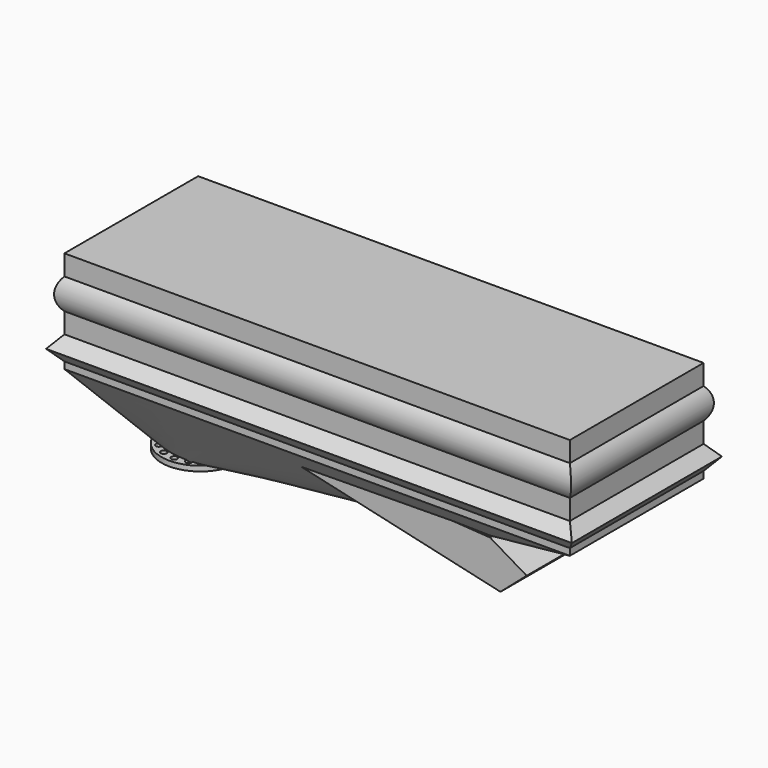
from build123d import *

# Parameters (mm, degrees)
F0_W       = 2580
F0_H       = 500
F1_DEPTH   = 475
F3_DEPTH   = 950
F5_DEPTH   = 2500
F1_FACE1_W = 2480
F1_FACE1_H = 820
F7_R       = 190
F7_R_2     = 15
F7_R_3     = 125
F9_DEPTH   = 25
F11_DEPTH  = 350


# Not quite as in the source:
# - the arcs of a loft's sections are written as splines that run evenly, so that the points pair up as in the source's solid


with BuildPart() as f1:
    # F0 (on Front) → F1 (new body, symmetric)
    with BuildSketch(Plane.XZ):
        Rectangle(F0_W, F0_H)
    extrude(amount=F1_DEPTH, both=True)

    # F2 (on face) → F3 (cut, through all)
    with BuildSketch(Plane.XZ.offset(475)):
        with BuildLine():
            Line((-1240, 150.2039159699), (-1240, 250))
            Line((-1240, 250), (-1240, 361.6854846478))
            Line((-1240, 361.6854846478), (-1458.3188199997, 361.6854846478))
            Line((-1458.3188199997, 361.6854846478), (-1458.3188199997, -342.266112566))
            Line((-1458.3188199997, -342.266112566), (-1240, -342.266112566))
            Line((-1240, -342.266112566), (-1240, -216.8733626604))
            Line((-1240, -216.8733626604), (-1290, -158.3347233453))
            Line((-1290, -158.3347233453), (-1240, -99.7960840301))
            Line((-1240, -99.7960840301), (-1240, 0))
            ThreePointArc((-1240, 0), (-1268.1875295389, 75.1019579849), (-1240, 150.2039159699))
        make_face()
        with BuildLine():
            ThreePointArc((1240, 150.2039159699), (1268.1875295389, 75.1019579849), (1240, 0))
            Line((1240, 0), (1240, -99.7960840301))
            Line((1240, -99.7960840301), (1290, -158.3347233453))
            Line((1290, -158.3347233453), (1240, -216.8733626604))
            Line((1240, -216.8733626604), (1240, -342.266112566))
            Line((1240, -342.266112566), (1458.3188199997, -342.266112566))
            Line((1458.3188199997, -342.266112566), (1458.3188199997, 361.6854846478))
            Line((1458.3188199997, 361.6854846478), (1240, 361.6854846478))
            Line((1240, 361.6854846478), (1240, 250))
            Line((1240, 250), (1240, 150.2039159699))
        make_face()
    extrude(amount=-F3_DEPTH, mode=Mode.SUBTRACT)

    # F4 (on Right) → F5 (cut, symmetric)
    with BuildSketch(Plane.YZ):
        with BuildLine():
            Line((-410, 150.2039159699), (-410, 250))
            Line((-410, 250), (-410, 357.733887434))
            Line((-410, 357.733887434), (-610, 357.733887434))
            Line((-610, 357.733887434), (-610, -342.266112566))
            Line((-610, -342.266112566), (-410, -342.266112566))
            Line((-410, -342.266112566), (-410, -216.8733626604))
            Line((-410, -216.8733626604), (-460, -158.3347233453))
            Line((-460, -158.3347233453), (-410, -99.7960840301))
            Line((-410, -99.7960840301), (-410, 0))
            ThreePointArc((-410, 0), (-438.1766354959, 75.1019579849), (-410, 150.2039159699))
        make_face()
        with BuildLine():
            ThreePointArc((410, 150.2039159699), (438.1766354959, 75.1019579849), (410, 0))
            Line((410, 0), (410, -99.7960840301))
            Line((410, -99.7960840301), (460, -158.3347233453))
            Line((460, -158.3347233453), (410, -216.8733626604))
            Line((410, -216.8733626604), (410, -342.266112566))
            Line((410, -342.266112566), (610, -342.266112566))
            Line((610, -342.266112566), (610, 357.733887434))
            Line((610, 357.733887434), (410, 357.733887434))
            Line((410, 357.733887434), (410, 250))
            Line((410, 250), (410, 150.2039159699))
        make_face()
    extrude(amount=F5_DEPTH, both=True, mode=Mode.SUBTRACT)

    # F7 (on offset) → F8 section 0
    with BuildSketch(Plane(origin=(0, 0, -650), x_dir=(1, 0, 0), z_dir=(0, 0, -1))):
        with BuildLine():
            add(Edge.make_bspline(
                [(-980.6526777918, 96.3350970343), (-986.9577951485, 91.1218414637), (-992.749308438, 85.2877302997), (-1003.0831296115, 72.6014268955), (-1007.6251819714, 65.749548349), (-1015.2854666523, 51.290980207), (-1018.4035095577, 43.6846481281), (-1023.0958773017, 28.0094499136), (-1024.6700861123, 19.9409713782), (-1026.2142118585, 3.6515321678), (-1026.1840906126, -4.5690257187), (-1024.5206344746, -20.8467119114), (-1022.8873407148, -28.9034377196), (-1018.080228379, -44.5438285428), (-1014.9065286684, -52.1271068182), (-1007.1404947661, -66.5291508238), (-1002.5483526049, -73.347560435), (-997.3350970343, -79.6526777918)],
                knots=[0, 0, 0, 0, 0.125, 0.125, 0.25, 0.25, 0.375, 0.375, 0.5, 0.5, 0.625, 0.625, 0.75, 0.75, 0.875, 0.875, 1, 1, 1, 1], degree=3))
            add(Edge.make_bspline(
                [(-997.3350970343, -79.6526777918), (-992.1218414637, -85.9577951485), (-986.2877302997, -91.749308438), (-973.6014268955, -102.0831296115), (-966.749548349, -106.6251819714), (-952.290980207, -114.2854666523), (-944.6846481281, -117.4035095577), (-929.0094499136, -122.0958773017), (-920.9409713782, -123.6700861123), (-904.6515321678, -125.2142118585), (-896.4309742813, -125.1840906126), (-880.1532880886, -123.5206344746), (-872.0965622804, -121.8873407148), (-856.4561714572, -117.080228379), (-848.8728931818, -113.9065286684), (-834.4708491762, -106.1404947661), (-827.652439565, -101.5483526049), (-821.3473222082, -96.3350970343)],
                knots=[0, 0, 0, 0, 0.125, 0.125, 0.25, 0.25, 0.375, 0.375, 0.5, 0.5, 0.625, 0.625, 0.75, 0.75, 0.875, 0.875, 1, 1, 1, 1], degree=3))
            add(Edge.make_bspline(
                [(-821.3473222082, -96.3350970343), (-815.0422048515, -91.1218414637), (-809.250691562, -85.2877302997), (-798.9168703885, -72.6014268955), (-794.3748180286, -65.749548349), (-786.7145333477, -51.290980207), (-783.5964904423, -43.6846481281), (-778.9041226983, -28.0094499136), (-777.3299138877, -19.9409713782), (-775.7857881415, -3.6515321678), (-775.8159093874, 4.5690257187), (-777.4793655254, 20.8467119114), (-779.1126592852, 28.9034377196), (-783.919771621, 44.5438285428), (-787.0934713316, 52.1271068182), (-794.8595052339, 66.5291508238), (-799.4516473951, 73.347560435), (-804.6649029657, 79.6526777918)],
                knots=[0, 0, 0, 0, 0.125, 0.125, 0.25, 0.25, 0.375, 0.375, 0.5, 0.5, 0.625, 0.625, 0.75, 0.75, 0.875, 0.875, 1, 1, 1, 1], degree=3))
            add(Edge.make_bspline(
                [(-804.6649029657, 79.6526777918), (-809.8781585363, 85.9577951485), (-815.7122697003, 91.749308438), (-828.3985731045, 102.0831296115), (-835.250451651, 106.6251819714), (-849.709019793, 114.2854666523), (-857.3153518719, 117.4035095577), (-872.9905500864, 122.0958773017), (-881.0590286218, 123.6700861123), (-897.3484678322, 125.2142118585), (-905.5690257187, 125.1840906126), (-921.8467119114, 123.5206344746), (-929.9034377196, 121.8873407148), (-945.5438285428, 117.080228379), (-953.1271068182, 113.9065286684), (-967.5291508238, 106.1404947661), (-974.347560435, 101.5483526049), (-980.6526777918, 96.3350970343)],
                knots=[0, 0, 0, 0, 0.125, 0.125, 0.25, 0.25, 0.375, 0.375, 0.5, 0.5, 0.625, 0.625, 0.75, 0.75, 0.875, 0.875, 1, 1, 1, 1], degree=3))
        make_face()
    # F1_face1 (on face) → F8 section 1
    with BuildSketch(Plane(origin=(0, 0, -250), x_dir=(1, 0, 0), z_dir=(0, 0, -1))):
        Rectangle(F1_FACE1_W, F1_FACE1_H)
    loft(ruled=True)

    # F10 (on Front) → F11 (join, symmetric)
    with BuildSketch(Plane.XZ):
        Polygon((980.0000190735, -444.9000358582), (800.8000254631, -338.5000228882), (-487.2000217438, -251.700013876), (851.3677120209, -556.3215613365), align=None)
    extrude(amount=F11_DEPTH, both=True)


with BuildPart() as f9:
    # F7 (on offset) → F9 (new body)
    with BuildSketch(Plane(origin=(0, 0, -650), x_dir=(1, 0, 0), z_dir=(0, 0, -1))):
        with Locations((-901, 0)):
            Circle(F7_R)
        with Locations((-1014.1370849898, -113.1370849898)):
            Circle(F7_R_2, mode=Mode.SUBTRACT)
        with Locations((-962.2293491784, -147.8207252018)):
            Circle(F7_R_2, mode=Mode.SUBTRACT)
        with Locations((-1048.8207252018, -61.2293491784)):
            Circle(F7_R_2, mode=Mode.SUBTRACT)
        with Locations((-901, -160)):
            Circle(F7_R_2, mode=Mode.SUBTRACT)
        with Locations((-839.7706508216, -147.8207252018)):
            Circle(F7_R_2, mode=Mode.SUBTRACT)
        with Locations((-787.8629150102, -113.1370849898)):
            Circle(F7_R_2, mode=Mode.SUBTRACT)
        with Locations((-753.1792747982, -61.2293491784)):
            Circle(F7_R_2, mode=Mode.SUBTRACT)
        with Locations((-1061, 0)):
            Circle(F7_R_2, mode=Mode.SUBTRACT)
        with Locations((-1048.8207252018, 61.2293491784)):
            Circle(F7_R_2, mode=Mode.SUBTRACT)
        with Locations((-1014.1370849898, 113.1370849898)):
            Circle(F7_R_2, mode=Mode.SUBTRACT)
        with Locations((-962.2293491784, 147.8207252018)):
            Circle(F7_R_2, mode=Mode.SUBTRACT)
        with Locations((-901, 0)):
            Circle(F7_R_3, mode=Mode.SUBTRACT)
        with Locations((-741, 0)):
            Circle(F7_R_2, mode=Mode.SUBTRACT)
        with Locations((-753.1792747982, 61.2293491784)):
            Circle(F7_R_2, mode=Mode.SUBTRACT)
        with Locations((-901, 160)):
            Circle(F7_R_2, mode=Mode.SUBTRACT)
        with Locations((-839.7706508216, 147.8207252018)):
            Circle(F7_R_2, mode=Mode.SUBTRACT)
        with Locations((-787.8629150102, 113.1370849898)):
            Circle(F7_R_2, mode=Mode.SUBTRACT)
    extrude(amount=-F9_DEPTH)


with BuildPart() as f12_1:
    # F12: copy of F9
    add(f9.part)


solid = Compound([f1.part, f12_1.part])
